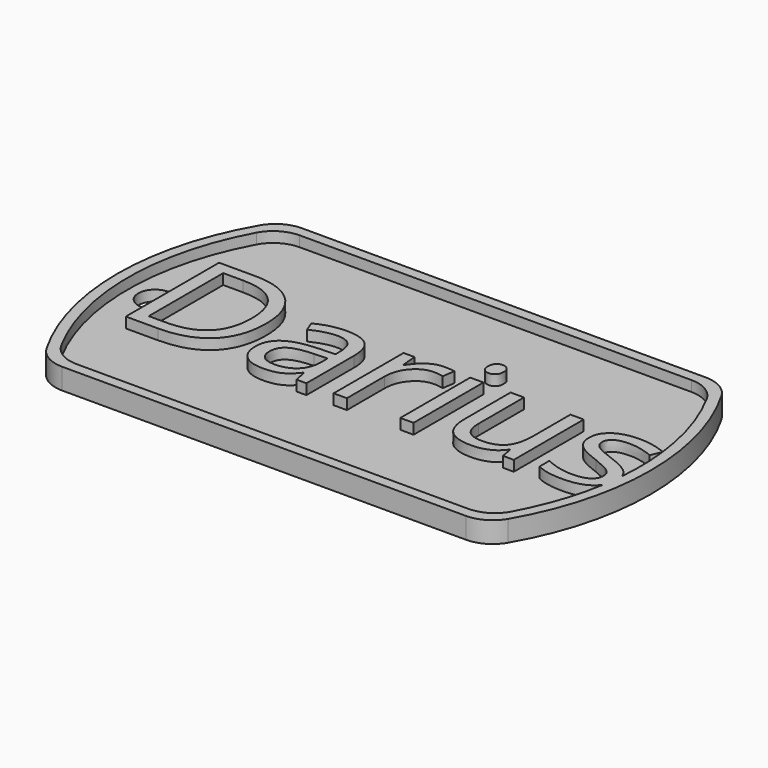
from build123d import *

# Parameters (mm, degrees)
F1_DEPTH     = 1
F3_DEPTH     = 1
F4_R         = 1.5875
F5_DEPTH     = 1
F6_TEXT_SIZE = 15.5596858046
F7_DEPTH     = 1


# Not quite as in the source:
# - Text() gives the source's letters only with a copy of the font that has no kerning and outlines rounded to 1/6400 em; it was checked with that copy


with BuildPart() as f1:
    # F0 (on Top) → F1 (new body)
    with BuildSketch(Plane.XY):
        with BuildLine():
            ThreePointArc((-19.2474145991, 14.2875), (-20.8349145991, 13.862130657), (-21.9970452561, 12.7))
            ThreePointArc((-21.9970452561, 12.7), (-25.4, 0), (-21.9970452561, -12.7))
            ThreePointArc((-21.9970452561, -12.7), (-20.8349145991, -13.862130657), (-19.2474145991, -14.2875))
            Line((-19.2474145991, -14.2875), (19.2474145991, -14.2875))
            ThreePointArc((19.2474145991, -14.2875), (20.8349145991, -13.862130657), (21.9970452561, -12.7))
            ThreePointArc((21.9970452561, -12.7), (25.4, 0), (21.9970452561, 12.7))
            ThreePointArc((21.9970452561, 12.7), (20.8349145991, 13.862130657), (19.2474145991, 14.2875))
            Line((19.2474145991, 14.2875), (-19.2474145991, 14.2875))
        make_face()
    extrude(amount=F1_DEPTH)

    # F2 (on face) → F3 (join)
    with BuildSketch(Plane.XY.offset(1)):
        with BuildLine():
            Line((19.2474145991, 14.2875), (-19.2474145991, 14.2875))
            ThreePointArc((-19.2474145991, 14.2875), (-20.8349145991, 13.862130657), (-21.9970452561, 12.7))
            ThreePointArc((-21.9970452561, 12.7), (-25.4, 0), (-21.9970452561, -12.7))
            ThreePointArc((-21.9970452561, -12.7), (-20.8349145991, -13.862130657), (-19.2474145991, -14.2875))
            Line((-19.2474145991, -14.2875), (19.2474145991, -14.2875))
            ThreePointArc((19.2474145991, -14.2875), (20.8349145991, -13.862130657), (21.9970452561, -12.7))
            ThreePointArc((21.9970452561, -12.7), (25.4, 0), (21.9970452561, 12.7))
            ThreePointArc((21.9970452561, 12.7), (20.8349145991, 13.862130657), (19.2474145991, 14.2875))
        make_face()
        with BuildLine():
            ThreePointArc((-21.4526124879, 11.6252061249), (-20.2856017842, 12.8404540819), (-18.6611352482, 13.2875))
            Line((-18.6611352482, 13.2875), (18.6611352482, 13.2875))
            ThreePointArc((18.6611352482, 13.2875), (20.2856017842, 12.8404540819), (21.4526124879, 11.6252061249))
            ThreePointArc((21.4526124879, 11.6252061249), (24.4, 0), (21.4526124879, -11.6252061249))
            ThreePointArc((21.4526124879, -11.6252061249), (20.2856017842, -12.8404540819), (18.6611352482, -13.2875))
            Line((18.6611352482, -13.2875), (-18.6611352482, -13.2875))
            ThreePointArc((-18.6611352482, -13.2875), (-20.2856017842, -12.8404540819), (-21.4526124879, -11.6252061249))
            ThreePointArc((-21.4526124879, -11.6252061249), (-24.4, 0), (-21.4526124879, 11.6252061249))
        make_face(mode=Mode.SUBTRACT)
    extrude(amount=F3_DEPTH)

    # F4 (on face) → F5 (cut)
    with BuildSketch(Plane.XY.offset(1)):
        with Locations((-21.821282804, 0)):
            Circle(F4_R)
    extrude(amount=-F5_DEPTH, mode=Mode.SUBTRACT)

    # F6 (on face) → F7 (join)
    with BuildSketch(Plane.XY.offset(1)):
        with Locations((-22.1229358576, -5.0110402517)):
            Text('Darius', F6_TEXT_SIZE, font='Open Sans', text_align=(TextAlign.LEFT, TextAlign.BOTTOM))
    extrude(amount=F7_DEPTH)


solid = f1.part
